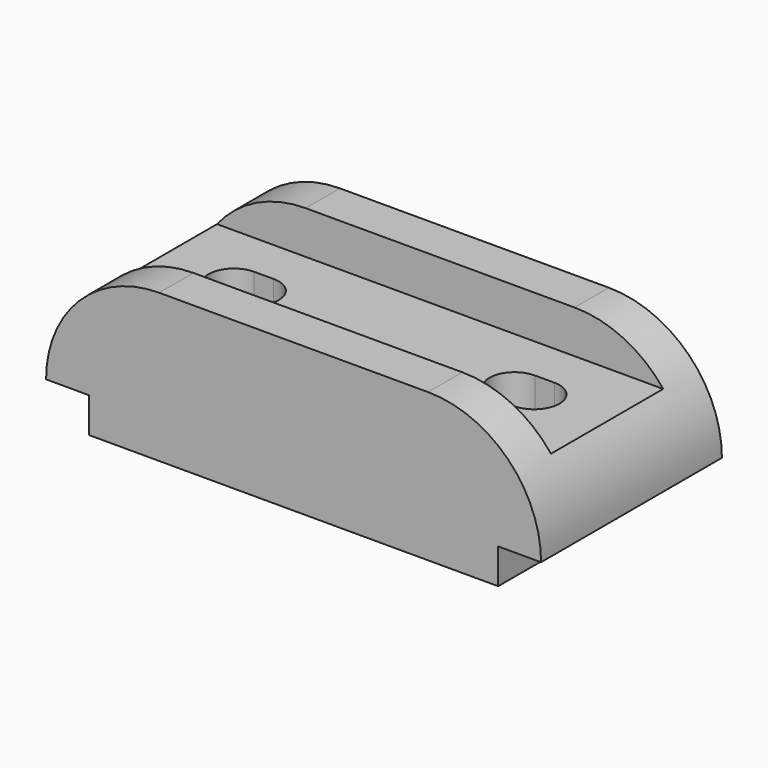
from build123d import *

# Parameters (mm, degrees)
F1_DEPTH      = 58
F2_W          = 36
F2_H          = 11
F3_DEPTH      = 63.501
F3_DEPTH_BACK = 63.501
F5_DEPTH      = 38.001


with BuildPart() as f1:
    # F0 (on Front) → F1 (new body)
    with BuildSketch(Plane.XZ):
        with BuildLine():
            Line((-52.5, 9), (-52.5, 0))
            Line((-52.5, 0), (52.5, 0))
            Line((52.5, 0), (52.5, 9))
            Line((52.5, 9), (63.5, 9))
            ThreePointArc((63.5, 9), (55.0060966544, 29.5060966544), (34.5, 38))
            Line((34.5, 38), (-34.5, 38))
            ThreePointArc((-34.5, 38), (-55.0060966544, 29.5060966544), (-63.5, 9))
            Line((-63.5, 9), (-52.5, 9))
        make_face()
    extrude(amount=-F1_DEPTH)

    # F2 (on Right) → F3 (cut, two sides)
    with BuildSketch(Plane.YZ) as f3_sk:
        with Locations((29, 32.5)):
            Rectangle(F2_W, F2_H)
    extrude(amount=-F3_DEPTH, mode=Mode.SUBTRACT)
    extrude(f3_sk.sketch, amount=F3_DEPTH_BACK, mode=Mode.SUBTRACT)

    # F4 (on Top) → F5 (cut, through all)
    with BuildSketch(Plane.XY):
        with BuildLine():
            Line((-33.5, 35.5), (-38.5, 35.5))
            ThreePointArc((-38.5, 35.5), (-45, 29), (-38.5, 22.5))
            Line((-38.5, 22.5), (-33.5, 22.5))
            ThreePointArc((-33.5, 22.5), (-27, 29), (-33.5, 35.5))
        make_face()
        with BuildLine():
            Line((38.5, 35.5), (33.5, 35.5))
            ThreePointArc((33.5, 35.5), (27, 29), (33.5, 22.5))
            Line((33.5, 22.5), (38.5, 22.5))
            ThreePointArc((38.5, 22.5), (45, 29), (38.5, 35.5))
        make_face()
    extrude(amount=F5_DEPTH, mode=Mode.SUBTRACT)


solid = f1.part
